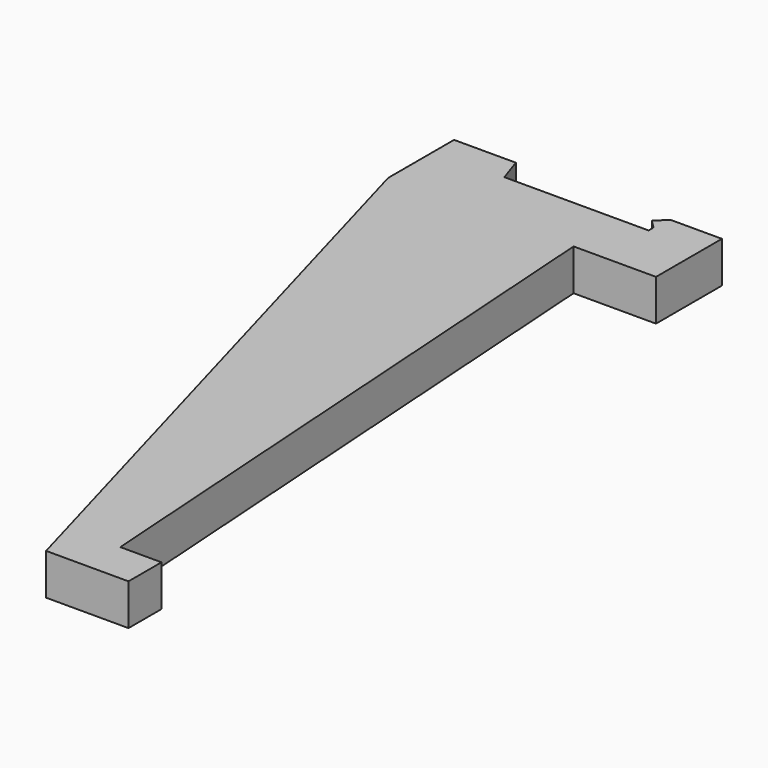
from build123d import *

# Parameters (mm, degrees)
F1_DEPTH = 10
F2_SIZE  = 1.99999
F3_SIZE  = 2.5


# Not quite as in the source:
# - a fillet or chamfer is up to 0.001 mm smaller than in the source, because OpenCascade refuses the exact size


with BuildPart() as f1:
    # F0 (on Top) → F1 (new body)
    with BuildSketch(Plane.XY):
        Polygon((35, 0), (0, 0), (-2, 6), (-17, 6), (-17, -14), (28, -14), (48, -14), (48, 6), (33, 6), (33, 1.5), (35, 1.5), align=None)
        Polygon((28, -14), (-17, -14), (28, -174), (48, -174), (48, -164), (38, -164), align=None)
    extrude(amount=F1_DEPTH)

    # F2 (size 2 in the source; OpenCascade refuses exactly that, so slightly less here)
    f2_edges = [f1.edges().sort_by_distance(p)[0] for p in [
        (33, 1.5, 5),
    ]]
    chamfer(f2_edges, length=F2_SIZE)

    # F3
    f3_edges = [f1.edges().sort_by_distance(p)[0] for p in [
        (33, 6, 5),
    ]]
    chamfer(f3_edges, length=F3_SIZE)


solid = f1.part
